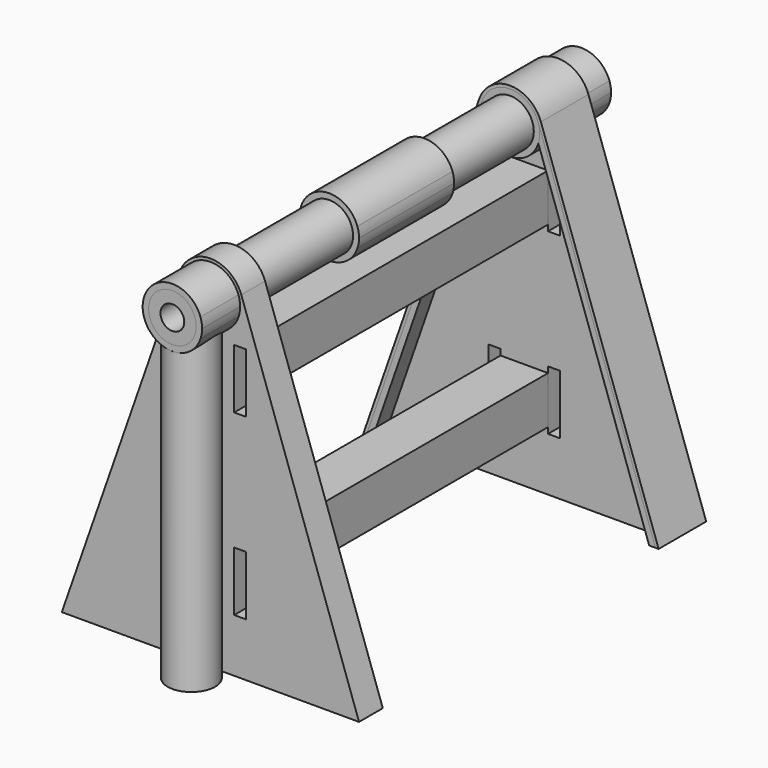
from build123d import *

# Parameters (mm, degrees)
F2_START  = 12
F1_W      = 8
F1_H      = 8
F1_W_2    = 6
F1_H_2    = 6
F2_DEPTH  = 61
F0_R      = 4
F0_R_2    = 2
F3_DEPTH  = 50
F4_DEPTH  = 55
F1_R      = 4
F1_R_2    = 3
F1_R_3    = 2
F5_DEPTH  = 120
F6_DEPTH  = 15
F7_START  = 73
F7_DEPTH  = 13
F8_DEPTH  = 86
F9_START  = 8
F9_DEPTH  = 4
F10_START = 73
F10_DEPTH = 5
F11_START = 33
F11_DEPTH = 20
F12_START = 5
F12_DEPTH = 10
F13_START = 5
F13_DEPTH = 10


# Not quite as in the source:
# - a feature names something its author has since deleted; it is built from what else it names


with BuildPart() as f2:
    # F1 (on Front) → F2 (new body)
    with BuildSketch(Plane.XZ.offset(F2_START)):
        with Locations((0, 44)):
            Rectangle(F1_W, F1_H)
        with Locations((0, 44)):
            Rectangle(F1_W_2, F1_H_2, mode=Mode.SUBTRACT)
    extrude(amount=F2_DEPTH)

    # F0 (on Top) → F3 (cut)
    with BuildSketch(Plane.XY):
        with Locations((0, -4)):
            Circle(F0_R)
        with Locations((0, -4)):
            Circle(F0_R_2, mode=Mode.SUBTRACT)
        with Locations((0, -82)):
            Circle(F0_R)
        with Locations((0, -82)):
            Circle(F0_R_2, mode=Mode.SUBTRACT)
        with Locations((0, -4)):
            Circle(F0_R_2)
        with Locations((0, -82)):
            Circle(F0_R_2)
    extrude(amount=F3_DEPTH, mode=Mode.SUBTRACT)


with BuildPart() as f2b:
    # F1 (on Front) → F2, piece 2 (new body)
    with BuildSketch(Plane.XZ.offset(F2_START)):
        with Locations((0, 14)):
            Rectangle(F1_W, F1_H)
        with Locations((0, 14)):
            Rectangle(F1_W_2, F1_H_2, mode=Mode.SUBTRACT)
    extrude(amount=F2_DEPTH)


with BuildPart() as f4:
    # F0 (on Top) → F4 (new body)
    with BuildSketch(Plane.XY):
        with Locations((0, -4)):
            Circle(F0_R)
        with Locations((0, -4)):
            Circle(F0_R_2, mode=Mode.SUBTRACT)
    extrude(amount=F4_DEPTH)


with BuildPart() as f4b:
    # F0 (on Top) → F4, piece 2 (new body)
    with BuildSketch(Plane.XY):
        with Locations((0, -82)):
            Circle(F0_R)
        with Locations((0, -82)):
            Circle(F0_R_2, mode=Mode.SUBTRACT)
    extrude(amount=F4_DEPTH)


with BuildPart() as f5_tool:
    # F1 (on Front) → F5 (new body)
    with BuildSketch(Plane.XZ):
        with BuildLine():
            ThreePointArc((4.7646536095, 53.4840593742), (4.9408130934, 54.2329498216), (5, 55))
            ThreePointArc((5, 55), (4.9298294248, 55.8347345938), (4.7212872631, 56.6460396651))
            ThreePointArc((4.7212872631, 56.6460396651), (0, 60), (-4.7212872631, 56.6460396651))
            ThreePointArc((-4.7212872631, 56.6460396651), (-4.9995298179, 55.0685682142), (-4.7646536095, 53.4840593742))
            ThreePointArc((-4.7646536095, 53.4840593742), (0, 50), (4.7646536095, 53.4840593742))
        make_face()
        with Locations((0, 55)):
            Circle(F1_R, mode=Mode.SUBTRACT)
        with Locations((0, 55)):
            Circle(F1_R)
        with Locations((0, 55)):
            Circle(F1_R_2, mode=Mode.SUBTRACT)
        with Locations((0, 55)):
            Circle(F1_R_2)
        with Locations((0, 55)):
            Circle(F1_R_3, mode=Mode.SUBTRACT)
        with Locations((0, 55)):
            Circle(F1_R_3)
    extrude(amount=F5_DEPTH)


with BuildPart() as f4_1:
    add(f4.part)

    # F5: cut by f5_tool
    add(f5_tool.part, mode=Mode.SUBTRACT)


with BuildPart() as f4b_1:
    add(f4b.part)

    # F5: cut by f5_tool
    add(f5_tool.part, mode=Mode.SUBTRACT)


with BuildPart() as f6:
    # F1 (on Front) → F6 (new body)
    with BuildSketch(Plane.XZ):
        with BuildLine():
            ThreePointArc((4.7646536095, 53.4840593742), (4.9408130934, 54.2329498216), (5, 55))
            ThreePointArc((5, 55), (4.9298294248, 55.8347345938), (4.7212872631, 56.6460396651))
            ThreePointArc((4.7212872631, 56.6460396651), (0, 60), (-4.7212872631, 56.6460396651))
            ThreePointArc((-4.7212872631, 56.6460396651), (-4.9995298179, 55.0685682142), (-4.7646536095, 53.4840593742))
            ThreePointArc((-4.7646536095, 53.4840593742), (0, 50), (4.7646536095, 53.4840593742))
        make_face()
        with Locations((0, 55)):
            Circle(F1_R, mode=Mode.SUBTRACT)
    extrude(amount=F6_DEPTH)


with BuildPart() as f7:
    # F1 (on Front) → F7 (new body)
    with BuildSketch(Plane.XZ.offset(F7_START)):
        with BuildLine():
            ThreePointArc((4.7646536095, 53.4840593742), (4.9408130934, 54.2329498216), (5, 55))
            ThreePointArc((5, 55), (4.9298294248, 55.8347345938), (4.7212872631, 56.6460396651))
            ThreePointArc((4.7212872631, 56.6460396651), (0, 60), (-4.7212872631, 56.6460396651))
            ThreePointArc((-4.7212872631, 56.6460396651), (-4.9995298179, 55.0685682142), (-4.7646536095, 53.4840593742))
            ThreePointArc((-4.7646536095, 53.4840593742), (0, 50), (4.7646536095, 53.4840593742))
        make_face()
        with Locations((0, 55)):
            Circle(F1_R, mode=Mode.SUBTRACT)
    extrude(amount=F7_DEPTH)


with BuildPart() as f8:
    # F1 (on Front) → F8 (new body)
    with BuildSketch(Plane.XZ):
        with Locations((0, 55)):
            Circle(F1_R)
        with Locations((0, 55)):
            Circle(F1_R_2, mode=Mode.SUBTRACT)
        with Locations((0, 55)):
            Circle(F1_R_2)
        with Locations((0, 55)):
            Circle(F1_R_3, mode=Mode.SUBTRACT)
    extrude(amount=F8_DEPTH)


with BuildPart() as f9:
    # F1 (on Front) → F9 (new body)
    with BuildSketch(Plane.XZ.offset(F9_START)):
        with BuildLine():
            Line((23.4114501868, 0), (5.019762505, 52.7523380162))
            ThreePointArc((5.019762505, 52.7523380162), (0, 49.5), (-5.019762505, 52.7523380162))
            Line((-5.019762505, 52.7523380162), (-23.4114501868, 0))
            Line((-23.4114501868, 0), (23.4114501868, 0))
        make_face()
        Polygon((-4, 19), (-4, 18), (4, 18), (4, 19), (6, 19), (6, 9), (4, 9), (4, 10), (-4, 10), (-4, 9), (-6, 9), (-6, 19), align=None, mode=Mode.SUBTRACT)
        Polygon((-4, 49), (-4, 48), (4, 48), (4, 49), (6, 49), (6, 39), (4, 39), (4, 40), (-4, 40), (-4, 39), (-6, 39), (-6, 49), align=None, mode=Mode.SUBTRACT)
        with Locations((0, 44)):
            Rectangle(F1_W, F1_H)
        with Locations((0, 44)):
            Rectangle(F1_W_2, F1_H_2, mode=Mode.SUBTRACT)
        with Locations((0, 14)):
            Rectangle(F1_W, F1_H)
        with Locations((0, 14)):
            Rectangle(F1_W_2, F1_H_2, mode=Mode.SUBTRACT)
        with Locations((0, 44)):
            Rectangle(F1_W_2, F1_H_2)
        with Locations((0, 14)):
            Rectangle(F1_W_2, F1_H_2)
        with BuildLine():
            Line((5.019762505, 52.7523380162), (4.7646536095, 53.4840593742))
            ThreePointArc((4.7646536095, 53.4840593742), (0, 50), (-4.7646536095, 53.4840593742))
            Line((-4.7646536095, 53.4840593742), (-5.019762505, 52.7523380162))
            ThreePointArc((-5.019762505, 52.7523380162), (0, 49.5), (5.019762505, 52.7523380162))
        make_face()
    extrude(amount=F9_DEPTH)


with BuildPart() as f10:
    # F1 (on Front) → F10 (new body)
    with BuildSketch(Plane.XZ.offset(F10_START)):
        with BuildLine():
            Line((23.4114501868, 0), (5.019762505, 52.7523380162))
            ThreePointArc((5.019762505, 52.7523380162), (0, 49.5), (-5.019762505, 52.7523380162))
            Line((-5.019762505, 52.7523380162), (-23.4114501868, 0))
            Line((-23.4114501868, 0), (23.4114501868, 0))
        make_face()
        Polygon((-4, 19), (-4, 18), (4, 18), (4, 19), (6, 19), (6, 9), (4, 9), (4, 10), (-4, 10), (-4, 9), (-6, 9), (-6, 19), align=None, mode=Mode.SUBTRACT)
        Polygon((-4, 49), (-4, 48), (4, 48), (4, 49), (6, 49), (6, 39), (4, 39), (4, 40), (-4, 40), (-4, 39), (-6, 39), (-6, 49), align=None, mode=Mode.SUBTRACT)
        with Locations((0, 44)):
            Rectangle(F1_W, F1_H)
        with Locations((0, 44)):
            Rectangle(F1_W_2, F1_H_2, mode=Mode.SUBTRACT)
        with Locations((0, 14)):
            Rectangle(F1_W, F1_H)
        with Locations((0, 14)):
            Rectangle(F1_W_2, F1_H_2, mode=Mode.SUBTRACT)
        with BuildLine():
            ThreePointArc((-5.019762505, 52.7523380162), (-5.3185042582, 53.5987461132), (-5.4755973993, 54.482474039))
            Line((-5.4755973993, 54.482474039), (-24.4704833956, 0))
            Line((-24.4704833956, 0), (-23.4114501868, 0))
            Line((-23.4114501868, 0), (-5.019762505, 52.7523380162))
        make_face()
        with BuildLine():
            Line((24.4704833956, 0), (5.4755973993, 54.482474039))
            ThreePointArc((5.4755973993, 54.482474039), (5.3185042582, 53.5987461132), (5.019762505, 52.7523380162))
            Line((5.019762505, 52.7523380162), (23.4114501868, 0))
            Line((23.4114501868, 0), (24.4704833956, 0))
        make_face()
        with Locations((0, 44)):
            Rectangle(F1_W_2, F1_H_2)
        with Locations((0, 14)):
            Rectangle(F1_W_2, F1_H_2)
        with BuildLine():
            Line((-24.4704833956, 0), (-5.4755973993, 54.482474039))
            ThreePointArc((-5.4755973993, 54.482474039), (-5.4600416743, 55.661774066), (-5.1934159894, 56.8106436316))
            Line((-5.1934159894, 56.8106436316), (-25, 0))
            Line((-25, 0), (-24.4704833956, 0))
        make_face()
        with BuildLine():
            ThreePointArc((5.5, 55), (5.4938959626, 54.7409495188), (5.4755973993, 54.482474039))
            Line((5.4755973993, 54.482474039), (24.4704833956, 0))
            Line((24.4704833956, 0), (25, 0))
            Line((25, 0), (5.1934159894, 56.8106436316))
            ThreePointArc((5.1934159894, 56.8106436316), (5.4228123673, 55.9182080532), (5.5, 55))
        make_face()
        with BuildLine():
            ThreePointArc((-4.7212872631, 56.6460396651), (0, 60), (4.7212872631, 56.6460396651))
            Line((4.7212872631, 56.6460396651), (5.4755973993, 54.482474039))
            ThreePointArc((5.4755973993, 54.482474039), (5.4938959626, 54.7409495188), (5.5, 55))
            ThreePointArc((5.5, 55), (5.4228123673, 55.9182080532), (5.1934159894, 56.8106436316))
            ThreePointArc((5.1934159894, 56.8106436316), (0, 60.5), (-5.1934159894, 56.8106436316))
            ThreePointArc((-5.1934159894, 56.8106436316), (-5.4600416743, 55.661774066), (-5.4755973993, 54.482474039))
            Line((-5.4755973993, 54.482474039), (-4.7212872631, 56.6460396651))
        make_face()
        with BuildLine():
            Line((5.019762505, 52.7523380162), (4.7646536095, 53.4840593742))
            ThreePointArc((4.7646536095, 53.4840593742), (0, 50), (-4.7646536095, 53.4840593742))
            Line((-4.7646536095, 53.4840593742), (-5.019762505, 52.7523380162))
            ThreePointArc((-5.019762505, 52.7523380162), (0, 49.5), (5.019762505, 52.7523380162))
        make_face()
        with BuildLine():
            ThreePointArc((-4.7646536095, 53.4840593742), (-4.9995298179, 55.0685682142), (-4.7212872631, 56.6460396651))
            Line((-4.7212872631, 56.6460396651), (-5.4755973993, 54.482474039))
            ThreePointArc((-5.4755973993, 54.482474039), (-5.3185042582, 53.5987461132), (-5.019762505, 52.7523380162))
            Line((-5.019762505, 52.7523380162), (-4.7646536095, 53.4840593742))
        make_face()
        with BuildLine():
            ThreePointArc((4.7212872631, 56.6460396651), (4.9298294248, 55.8347345938), (5, 55))
            ThreePointArc((5, 55), (4.9408130934, 54.2329498216), (4.7646536095, 53.4840593742))
            Line((4.7646536095, 53.4840593742), (5.019762505, 52.7523380162))
            ThreePointArc((5.019762505, 52.7523380162), (5.3185042582, 53.5987461132), (5.4755973993, 54.482474039))
            Line((5.4755973993, 54.482474039), (4.7212872631, 56.6460396651))
        make_face()
    extrude(amount=F10_DEPTH)


with BuildPart() as f11:
    # F1 (on Front) → F11 (new body)
    with BuildSketch(Plane.XZ.offset(F11_START)):
        with BuildLine():
            ThreePointArc((4.7646536095, 53.4840593742), (4.9408130934, 54.2329498216), (5, 55))
            ThreePointArc((5, 55), (4.9298294248, 55.8347345938), (4.7212872631, 56.6460396651))
            ThreePointArc((4.7212872631, 56.6460396651), (0, 60), (-4.7212872631, 56.6460396651))
            ThreePointArc((-4.7212872631, 56.6460396651), (-4.9995298179, 55.0685682142), (-4.7646536095, 53.4840593742))
            ThreePointArc((-4.7646536095, 53.4840593742), (0, 50), (4.7646536095, 53.4840593742))
        make_face()
        with Locations((0, 55)):
            Circle(F1_R, mode=Mode.SUBTRACT)
    extrude(amount=F11_DEPTH)


with BuildPart() as f12:
    # F1 (on Front) → F12 (new body)
    with BuildSketch(Plane.XZ.offset(F12_START)):
        with BuildLine():
            ThreePointArc((-5.019762505, 52.7523380162), (-5.3185042582, 53.5987461132), (-5.4755973993, 54.482474039))
            Line((-5.4755973993, 54.482474039), (-24.4704833956, 0))
            Line((-24.4704833956, 0), (-23.4114501868, 0))
            Line((-23.4114501868, 0), (-5.019762505, 52.7523380162))
        make_face()
        with BuildLine():
            ThreePointArc((-4.7646536095, 53.4840593742), (-4.9995298179, 55.0685682142), (-4.7212872631, 56.6460396651))
            Line((-4.7212872631, 56.6460396651), (-5.4755973993, 54.482474039))
            ThreePointArc((-5.4755973993, 54.482474039), (-5.3185042582, 53.5987461132), (-5.019762505, 52.7523380162))
            Line((-5.019762505, 52.7523380162), (-4.7646536095, 53.4840593742))
        make_face()
    extrude(amount=F12_DEPTH)


with BuildPart() as f12b:
    # F1 (on Front) → F12, piece 2 (new body)
    with BuildSketch(Plane.XZ.offset(F12_START)):
        with BuildLine():
            Line((24.4704833956, 0), (5.4755973993, 54.482474039))
            ThreePointArc((5.4755973993, 54.482474039), (5.3185042582, 53.5987461132), (5.019762505, 52.7523380162))
            Line((5.019762505, 52.7523380162), (23.4114501868, 0))
            Line((23.4114501868, 0), (24.4704833956, 0))
        make_face()
        with BuildLine():
            ThreePointArc((4.7212872631, 56.6460396651), (4.9298294248, 55.8347345938), (5, 55))
            ThreePointArc((5, 55), (4.9408130934, 54.2329498216), (4.7646536095, 53.4840593742))
            Line((4.7646536095, 53.4840593742), (5.019762505, 52.7523380162))
            ThreePointArc((5.019762505, 52.7523380162), (5.3185042582, 53.5987461132), (5.4755973993, 54.482474039))
            Line((5.4755973993, 54.482474039), (4.7212872631, 56.6460396651))
        make_face()
    extrude(amount=F12_DEPTH)


with BuildPart() as f13:
    # F1 (on Front) → F13 (new body)
    with BuildSketch(Plane.XZ.offset(F13_START)):
        with BuildLine():
            ThreePointArc((5.5, 55), (5.4938959626, 54.7409495188), (5.4755973993, 54.482474039))
            Line((5.4755973993, 54.482474039), (24.4704833956, 0))
            Line((24.4704833956, 0), (25, 0))
            Line((25, 0), (5.1934159894, 56.8106436316))
            ThreePointArc((5.1934159894, 56.8106436316), (5.4228123673, 55.9182080532), (5.5, 55))
        make_face()
        with BuildLine():
            ThreePointArc((-4.7212872631, 56.6460396651), (0, 60), (4.7212872631, 56.6460396651))
            Line((4.7212872631, 56.6460396651), (5.4755973993, 54.482474039))
            ThreePointArc((5.4755973993, 54.482474039), (5.4938959626, 54.7409495188), (5.5, 55))
            ThreePointArc((5.5, 55), (5.4228123673, 55.9182080532), (5.1934159894, 56.8106436316))
            ThreePointArc((5.1934159894, 56.8106436316), (0, 60.5), (-5.1934159894, 56.8106436316))
            ThreePointArc((-5.1934159894, 56.8106436316), (-5.4600416743, 55.661774066), (-5.4755973993, 54.482474039))
            Line((-5.4755973993, 54.482474039), (-4.7212872631, 56.6460396651))
        make_face()
        with BuildLine():
            Line((-24.4704833956, 0), (-5.4755973993, 54.482474039))
            ThreePointArc((-5.4755973993, 54.482474039), (-5.4600416743, 55.661774066), (-5.1934159894, 56.8106436316))
            Line((-5.1934159894, 56.8106436316), (-25, 0))
            Line((-25, 0), (-24.4704833956, 0))
        make_face()
    extrude(amount=F13_DEPTH)


solid = Compound([f2.part, f2b.part, f4_1.part, f4b_1.part, f6.part, f7.part, f8.part, f9.part, f10.part, f11.part, f12.part, f12b.part, f13.part])
